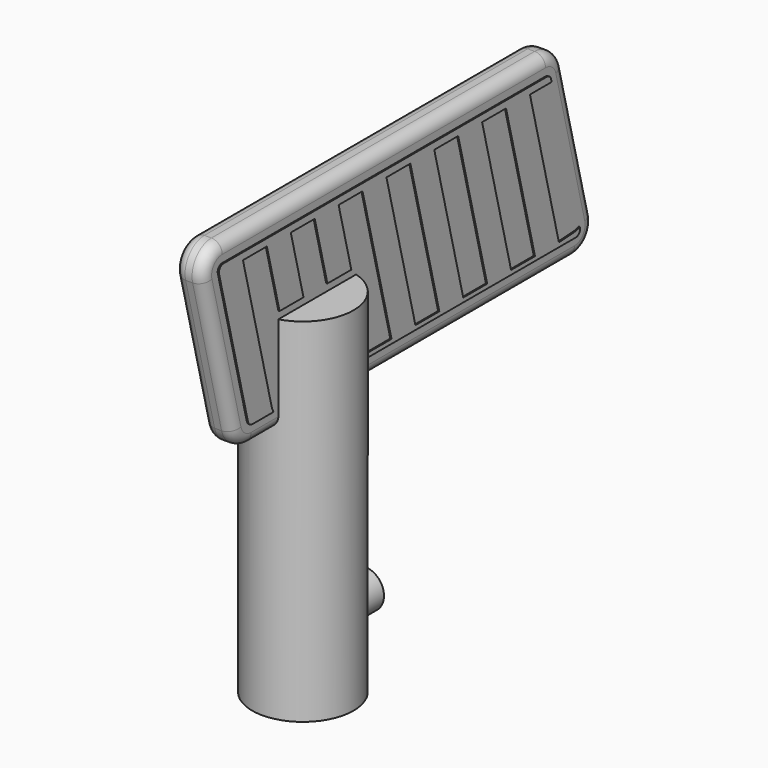
from build123d import *

# Parameters (mm, degrees)
F0_R      = 5.334
F1_DEPTH  = 37.084
F2_R      = 2.032
F3_DEPTH  = 8.128
F4_W      = 3.0226
F4_H      = 47.752
F5_DEPTH  = 10.16
F7_DEPTH  = 3.0226
F9_DEPTH  = 3.0226
F10_R     = 2.54
F11_R     = 1.143
F13_DEPTH = 0.127


# Not quite as in the source:
# - a feature of the source that left no trace in its solid (it failed there, or was rolled back) is left out


with BuildPart() as f1:
    # F0 (on Top) → F1 (new body)
    with BuildSketch(Plane.XY):
        Circle(F0_R)
    extrude(amount=F1_DEPTH)

    # F2 (on Front) → F3 (join)
    with BuildSketch(Plane.XZ):
        with Locations((0, 6.2738)):
            Circle(F2_R)
    extrude(amount=-F3_DEPTH)

    # F4 (on face) → F5 (join, symmetric)
    with BuildSketch(Plane.XY.offset(37.084)):
        with Locations((0, 13.208)):
            Rectangle(F4_W, F4_H)
    extrude(amount=F5_DEPTH, both=True)

    # F6 (on face) → F7 (join)
    with BuildSketch(Plane(origin=(-1.5113, 0, 0), x_dir=(0, -1, 0), z_dir=(-1, 0, 0))):
        Polygon((15.748, 47.244), (10.668, 47.244), (10.668, 26.924), align=None)
        Polygon((-37.084, 47.244), (-37.084, 26.924), (-32.004, 47.244), align=None)
    extrude(amount=-F7_DEPTH)

    # F8 (on face) → F9 (cut, through all)
    with BuildSketch(Plane(origin=(-1.5113, 0, 0), x_dir=(0, -1, 0), z_dir=(-1, 0, 0))):
        Polygon((-37.084, 47.244), (-37.084, 26.924), (-32.004, 47.244), align=None)
    extrude(amount=-F9_DEPTH, mode=Mode.SUBTRACT)

    # F10
    f10_edges = [f1.edges().sort_by_distance(p)[0] for p in [
        (0, 32.004, 47.244),
        (0, 37.084, 26.924),
        (0, -15.748, 47.244),
        (0, -10.668, 26.924),
    ]]
    fillet(f10_edges, radius=F10_R)

    # F11
    f11_edges = [f1.edges().sort_by_distance(p)[0] for p in [
        (-1.5113, 8.763, 47.244),
        (1.5113, 8.763, 47.244),
        (-1.5113, 34.38999, 37.70004),
        (1.5113, 34.38999, 37.70004),
        (1.5113, 31.583975, 46.706042),
        (-1.5113, 31.583975, 46.706042),
        (-1.5113, 35.83287, 27.900853),
        (1.5113, 35.83287, 27.900853),
        (1.5113, 19.473124, 26.924),
        (-1.5113, 19.473124, 26.924),
        (1.5113, -14.49687, 46.267147),
        (1.5113, -13.05399, 36.46796),
        (-1.5113, -14.49687, 46.267147),
        (-1.5113, -13.05399, 36.46796),
        (1.5113, -10.247975, 27.461958),
        (1.5113, -6.900124, 26.924),
        (-1.5113, -6.900124, 26.924),
        (-1.5113, -10.247975, 27.461958),
    ]]
    fillet(f11_edges, radius=F11_R)

    # F12 (on face) → F13 (join)
    with BuildSketch(Plane.YZ.offset(1.5113)):
        with BuildLine():
            Line((-6.1186332318, 29.319293674), (-9.2636532318, 29.319293674))
            ThreePointArc((-9.2636532318, 29.319293674), (-9.0520071402, 28.9937255277), (-8.6848279277, 28.8673605332))
            Line((-8.6848279277, 28.8673605332), (-5.9157811718, 28.8673605332))
            Line((-5.9157811718, 28.8673605332), (-6.1186332318, 29.319293674))
        make_face()
        Polygon((-9.9286332318, 44.559293674), (-13.0736532318, 44.559293674), (-9.2636532318, 29.319293674), (-6.1186332318, 29.319293674), align=None)
        Polygon((-3.6385932318, 44.559293674), (-6.7836132318, 44.559293674), (-5.1148799466, 37.8843605332), (-1.9698599466, 37.8843605332), align=None)
        Polygon((2.6514467682, 44.559293674), (-0.4935732318, 44.559293674), (1.1751600534, 37.8843605332), (4.3201800534, 37.8843605332), align=None)
        with BuildLine():
            ThreePointArc((33.8308279277, 28.8673605332), (34.3011024, 29.0968207875), (34.4096532318, 29.608706326))
            Line((34.4096532318, 29.608706326), (33.8308279277, 29.464))
            Line((33.8308279277, 29.464), (31.6216067682, 29.319293674))
            Line((31.6216067682, 29.319293674), (28.4765867682, 29.319293674))
            Line((28.4765867682, 29.319293674), (25.3315667682, 29.319293674))
            Line((25.3315667682, 29.319293674), (22.1865467682, 29.319293674))
            Line((22.1865467682, 29.319293674), (19.0415267682, 29.319293674))
            Line((19.0415267682, 29.319293674), (15.8965067682, 29.319293674))
            Line((15.8965067682, 29.319293674), (12.7514867682, 29.319293674))
            Line((12.7514867682, 29.319293674), (9.6064667682, 29.319293674))
            Line((9.6064667682, 29.319293674), (6.4614467682, 29.319293674))
            Line((6.4614467682, 29.319293674), (5.9157811718, 31.5019560598))
            Line((5.9157811718, 31.5019560598), (5.9157811718, 28.8673605332))
            Line((5.9157811718, 28.8673605332), (33.8308279277, 28.8673605332))
        make_face()
        with BuildLine():
            ThreePointArc((-12.4948279277, 45.3006394668), (-12.9651024, 45.0711792125), (-13.0736532318, 44.559293674))
            Line((-13.0736532318, 44.559293674), (-9.9286332318, 44.559293674))
            Line((-9.9286332318, 44.559293674), (-6.7836132318, 44.559293674))
            Line((-6.7836132318, 44.559293674), (-3.6385932318, 44.559293674))
            Line((-3.6385932318, 44.559293674), (-0.4935732318, 44.559293674))
            Line((-0.4935732318, 44.559293674), (2.6514467682, 44.559293674))
            Line((2.6514467682, 44.559293674), (5.7964667682, 44.559293674))
            Line((5.7964667682, 44.559293674), (8.9414867682, 44.559293674))
            Line((8.9414867682, 44.559293674), (12.0865067682, 44.559293674))
            Line((12.0865067682, 44.559293674), (15.2315267682, 44.559293674))
            Line((15.2315267682, 44.559293674), (18.3765467682, 44.559293674))
            Line((18.3765467682, 44.559293674), (21.5215667682, 44.559293674))
            Line((21.5215667682, 44.559293674), (24.6665867682, 44.559293674))
            Line((24.6665867682, 44.559293674), (27.8116067682, 44.559293674))
            Line((27.8116067682, 44.559293674), (30.6720063948, 44.559293674))
            Line((30.6720063948, 44.559293674), (30.5996532318, 44.848706326))
            ThreePointArc((30.5996532318, 44.848706326), (30.3880071402, 45.1742744723), (30.0208279277, 45.3006394668))
            Line((30.0208279277, 45.3006394668), (-12.4948279277, 45.3006394668))
        make_face()
        Polygon((8.9414867682, 44.559293674), (5.7964667682, 44.559293674), (9.6064667682, 29.319293674), (12.7514867682, 29.319293674), align=None)
        Polygon((15.2315267682, 44.559293674), (12.0865067682, 44.559293674), (15.8965067682, 29.319293674), (19.0415267682, 29.319293674), align=None)
        Polygon((25.3315667682, 29.319293674), (21.5215667682, 44.559293674), (18.3765467682, 44.559293674), (22.1865467682, 29.319293674), align=None)
        Polygon((31.6216067682, 29.319293674), (27.8116067682, 44.559293674), (24.6665867682, 44.559293674), (28.4765867682, 29.319293674), align=None)
    extrude(amount=F13_DEPTH)

    # F14: F1 across plane


with BuildPart() as f1_1:
    add(f1.part)
    add(f1.part.mirror(Plane.YZ))

    # F17: F1 across plane


with BuildPart() as f1_2:
    add(f1_1.part)
    add(f1_1.part.mirror(Plane.YZ))


solid = f1_2.part
